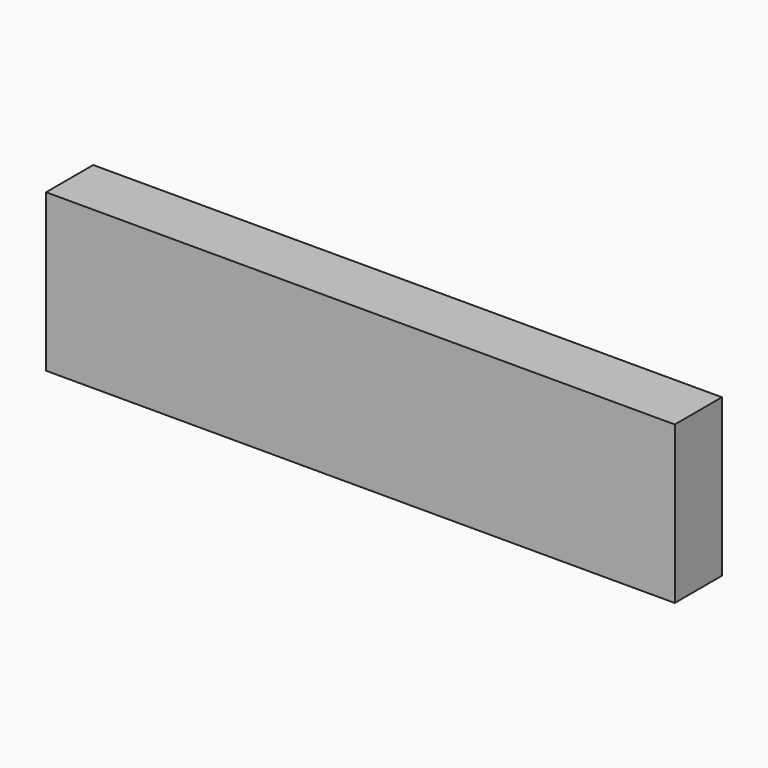
from build123d import *

# Parameters (mm, degrees)
F0_W     = 203.2
F0_H     = 50.8
F1_DEPTH = 19.05


# Not quite as in the source:
# - a length typed as a fraction of an inch, garbled in the dataset ("3 / 203.2 mm" for 3/8 in), is restored


with BuildPart() as f1:
    # F0 (on Front) → F1 (new body)
    with BuildSketch(Plane.XZ):
        with Locations((-56.1882283073, -5.475784809)):
            Rectangle(F0_W, F0_H)
    extrude(amount=F1_DEPTH)


solid = f1.part
